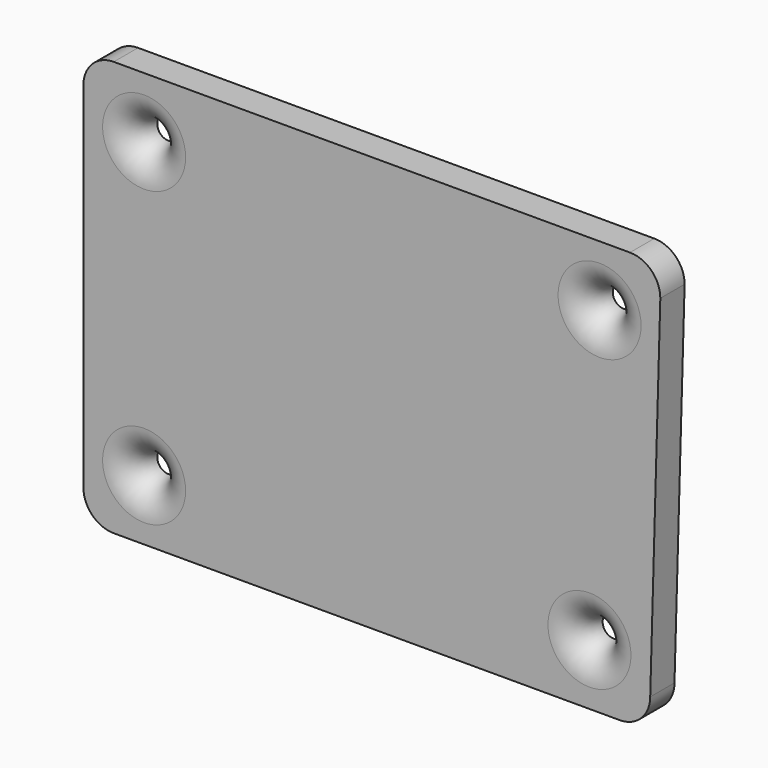
from build123d import *

# Parameters (mm, degrees)
F0_W     = 3.689654345
F0_H     = 2
F0_W_2   = 6
F0_H_2   = 6
F0_R     = 1.1
F0_W_3   = 3.6920479782
F0_W_4   = 3.5541171093
F1_DEPTH = 3
F2_R     = 2.99999


# Not quite as in the source:
# - a fillet or chamfer is up to 0.001 mm smaller than in the source, because OpenCascade refuses the exact size


with BuildPart() as f1:
    # F0 (on Front) → F1 (new body)
    with BuildSketch(Plane.XZ):
        with BuildLine():
            Line((25.5162836348, 23.2549019608), (-25.4837163652, 23.2549019608))
            ThreePointArc((-25.4837163652, 23.2549019608), (-27.6050367088, 22.3762223043), (-28.4837163652, 20.2549019608))
            Line((-28.4837163652, 20.2549019608), (-28.4837163652, -14.7450980392))
            ThreePointArc((-28.4837163652, -14.7450980392), (-27.6050367088, -16.8664183828), (-25.4837163652, -17.7450980392))
            Line((-25.4837163652, -17.7450980392), (24.5162836348, -17.7450980392))
            ThreePointArc((24.5162836348, -17.7450980392), (26.6376039783, -16.8664183828), (27.5162836348, -14.7450980392))
            Line((27.5162836348, -14.7450980392), (28.5162836348, 20.2549019608))
            ThreePointArc((28.5162836348, 20.2549019608), (27.6376039783, 22.3762223043), (25.5162836348, 23.2549019608))
        make_face()
        Polygon((-25.4837163652, -8.7450980392), (-25.4837163652, -6.7450980392), (-25.4837163652, -4.7450980392), (-25.4837163652, -2.7450980392), (-25.4837163652, -0.7450980392), (-25.4837163652, 14.2549019608), (-25.4837163652, 20.2549019608), (-19.4837163652, 20.2549019608), (19.5162836348, 20.2549019608), (25.5162836348, 20.2549019608), (25.5162836348, 14.2549019608), (25.5162836348, -14.7450980392), (24.5162836348, -14.7450980392), (18.5162836348, -14.7450980392), (-19.4837163652, -14.7450980392), (-25.4837163652, -14.7450980392), align=None, mode=Mode.SUBTRACT)
        Polygon((-21.929599256, -6.7450980392), (-25.4837163652, -6.7450980392), (-25.4837163652, -8.7450980392), (-19.4837163652, -8.7450980392), (-19.4837163652, -14.7450980392), (18.5162836348, -14.7450980392), (18.5162836348, -8.7450980392), (24.5162836348, -8.7450980392), (24.5162836348, -14.7450980392), (25.5162836348, -14.7450980392), (25.5162836348, 14.2549019608), (19.5162836348, 14.2549019608), (19.5162836348, 20.2549019608), (-19.4837163652, 20.2549019608), (-19.4837163652, 14.2549019608), (-25.4837163652, 14.2549019608), (-25.4837163652, -0.7450980392), (-21.791668387, -0.7450980392), (-21.791668387, -2.7450980392), (-25.4837163652, -2.7450980392), (-25.4837163652, -4.7450980392), (-21.929599256, -4.7450980392), align=None)
        with Locations((22.6714564623, -1.7450980392)):
            Rectangle(F0_W, F0_H, mode=Mode.SUBTRACT)
        with Locations((22.5162836348, 17.2549019608)):
            Rectangle(F0_W_2, F0_H_2)
        with Locations((22.5162836348, 17.2549019608)):
            Circle(F0_R, mode=Mode.SUBTRACT)
        with Locations((-22.4837163652, 17.2549019608)):
            Rectangle(F0_W_2, F0_H_2)
        with Locations((-22.4837163652, 17.2549019608)):
            Circle(F0_R, mode=Mode.SUBTRACT)
        with Locations((-22.4837163652, -11.7450980392)):
            Rectangle(F0_W_2, F0_H_2)
        with Locations((-22.4837163652, -11.7450980392)):
            Circle(F0_R, mode=Mode.SUBTRACT)
        with Locations((21.5162836348, -11.7450980392)):
            Rectangle(F0_W_2, F0_H_2)
        with Locations((21.5162836348, -11.7450980392)):
            Circle(F0_R, mode=Mode.SUBTRACT)
        with Locations((-23.6376923761, -1.7450980392)):
            Rectangle(F0_W_3, F0_H)
        with Locations((22.6714564623, -1.7450980392)):
            Rectangle(F0_W, F0_H)
        with Locations((-23.7066578106, -5.7450980392)):
            Rectangle(F0_W_4, F0_H)
    extrude(amount=F1_DEPTH)

    # F2 (radius 3 in the source; OpenCascade refuses exactly that, so slightly less here)
    f2_edges = [f1.edges().sort_by_distance(p)[0] for p in [
        (-23.583716, -3, -11.745098),
        (-23.583716, -3, 17.254902),
        (21.416284, -3, 17.254902),
        (20.416284, -3, -11.745098),
    ]]
    fillet(f2_edges, radius=F2_R)


solid = f1.part
